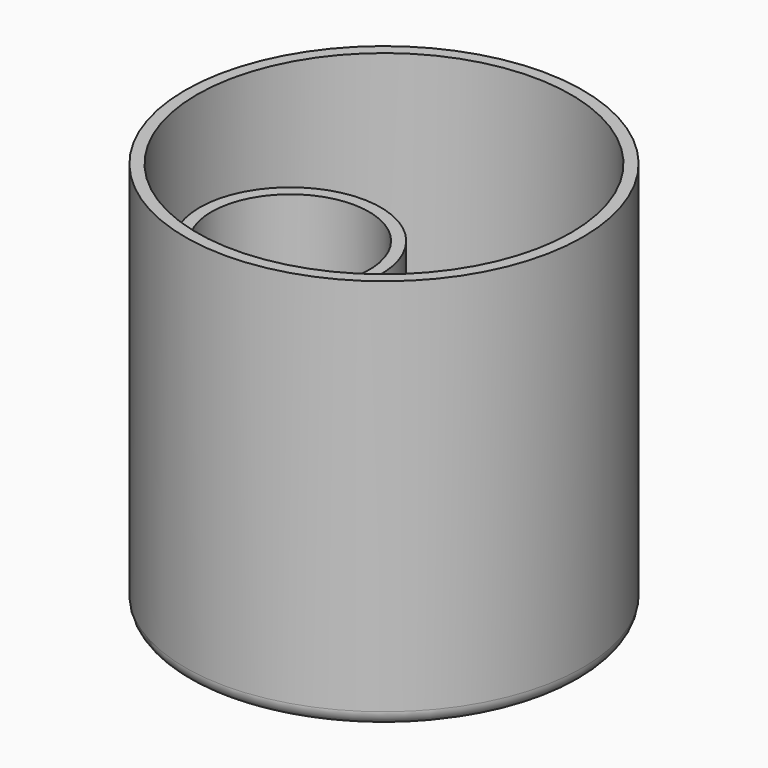
from build123d import *

# Parameters (mm, degrees)
F2_W     = 1.2
F2_H     = 30
F4_DEPTH = 12.5


# Not quite as in the source:
# - a fillet or chamfer that OpenCascade refuses, or shapes differently, is made with other operations: its cross-section is extruded or revolved along the edge and cut away or added


with BuildPart() as f1:
    # F0 (on Front) → F1 (revolve)
    with BuildSketch(Plane.XZ):
        Polygon((-20.2, 0), (0, 0), (0, 1), (-19, 1), (-19, 40), (-20.2, 40), align=None)
    revolve(axis=Axis((0, 0, 0.5), (0, 0, -1)))

    # F2 (on Front) → F3 (revolve)
    with BuildSketch(Plane.XZ):
        with Locations((-18.1225388443, 15)):
            Rectangle(F2_W, F2_H)
    revolve(axis=Axis((-9.5225388443, 0, 9.0516569445), (0, 0, -1)))

    # F4 (cut, symmetric): a face of the model
    f4_faces = [f1.faces().sort_by_distance(p)[0] for p in [
        (-9.5225388443, 0, 1),
    ]]
    extrude(f4_faces, amount=F4_DEPTH, both=True, mode=Mode.SUBTRACT)

    # F5: fillet of radius 1.5 on 4 edges, made by hand

    # F5_s1 → F5_t2 (revolve)
    with BuildSketch(Plane.XZ):
        with BuildLine():
            ThreePointArc((-17.5, 1), (-18.5606601718, 1.4393398282), (-19, 2.5))
            Line((-19, 2.5), (-19.03, 2.5))
            Line((-19.03, 2.5), (-19.03, 0.97))
            Line((-19.03, 0.97), (-17.5, 0.97))
            Line((-17.5, 0.97), (-17.5, 1))
        make_face()
    revolve(axis=Axis((0, 0, 1), (0, 0, -1)))

    # F5_s3 → F5_t4 (revolve)
    with BuildSketch(Plane.XZ):
        with BuildLine():
            ThreePointArc((-18.7225388443, 2.5), (-19.1618786725, 1.4393398282), (-20.2225388443, 1))
            Line((-20.2225388443, 1), (-20.2225388443, 0.97))
            Line((-20.2225388443, 0.97), (-18.6925388443, 0.97))
            Line((-18.6925388443, 0.97), (-18.6925388443, 2.5))
            Line((-18.6925388443, 2.5), (-18.7225388443, 2.5))
        make_face()
    revolve(axis=Axis((-9.5225388443, 0, 1), (0, 0, -1)))

    # F5_s5 → F5_t6 (revolve, cut)
    with BuildSketch(Plane.XZ):
        with BuildLine():
            ThreePointArc((-18.7, 0), (-19.7606601718, 0.4393398282), (-20.2, 1.5))
            Line((-20.2, 1.5), (-20.23, 1.5))
            Line((-20.23, 1.5), (-20.23, -0.03))
            Line((-20.23, -0.03), (-18.7, -0.03))
            Line((-18.7, -0.03), (-18.7, 0))
        make_face()
    revolve(axis=Axis((0, 0, 0), (0, 0, -1)), mode=Mode.SUBTRACT)

    # F5_s7 → F5_t8 (revolve, cut)
    with BuildSketch(Plane.XZ):
        with BuildLine():
            ThreePointArc((-19.0225388443, 0), (-17.9618786725, 0.4393398282), (-17.5225388443, 1.5))
            Line((-17.5225388443, 1.5), (-17.4925388443, 1.5))
            Line((-17.4925388443, 1.5), (-17.4925388443, -0.03))
            Line((-17.4925388443, -0.03), (-19.0225388443, -0.03))
            Line((-19.0225388443, -0.03), (-19.0225388443, 0))
        make_face()
    revolve(axis=Axis((-9.5225388443, 0, 0), (0, 0, 1)), mode=Mode.SUBTRACT)


solid = f1.part
